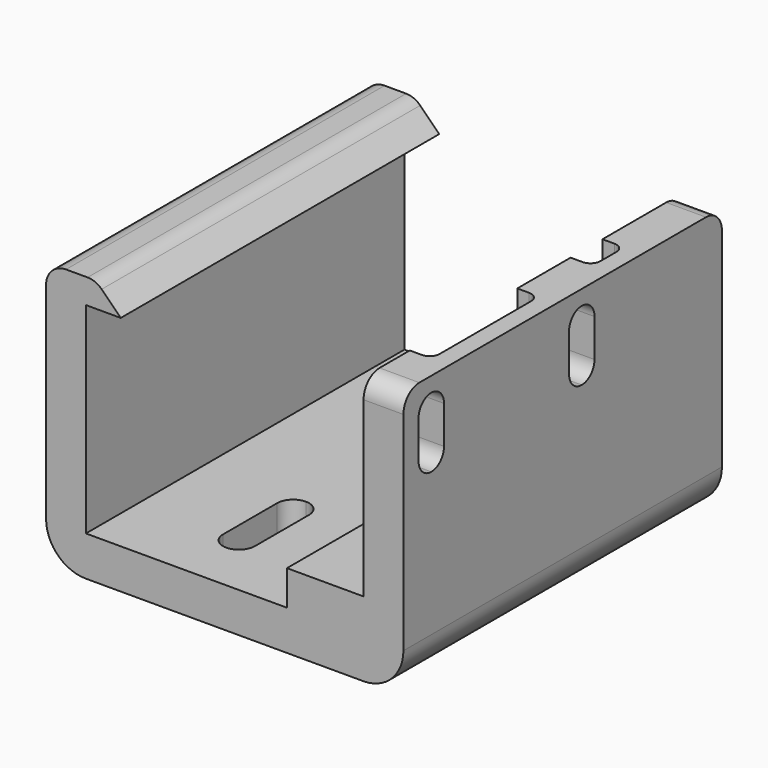
from build123d import *

# Parameters (mm, degrees)
F1_DEPTH  = 40
F2_R      = 4
F3_R      = 2
F4_W      = 3.2
F4_H      = 7
F5_DEPTH  = 4
F6_R      = 1.59999
F7_W      = 3.2
F7_H      = 10
F8_DEPTH  = 4
F9_R      = 1.59999
F10_W     = 2.2
F10_H     = 4
F10_H_2   = 13.5
F11_DEPTH = 17
F12_R     = 2
F13_R     = 1
F14_R     = 2


# Not quite as in the source:
# - a fillet or chamfer is up to 0.001 mm smaller than in the source, because OpenCascade refuses the exact size


with BuildPart() as f1:
    # F0 (on Front) → F1 (new body)
    with BuildSketch(Plane.XZ):
        Polygon((21.0562500745, -30.2744720221), (21.0562500745, -3.3744720221), (17.0562500745, -3.3744720221), (17.0562500745, -22.7744720221), (9.3562500745, -22.7744720221), (9.3562500745, -26.2744720221), (-10.8437499255, -26.2744720221), (-10.8437499255, -6.0744720221), (-7.3437499255, -6.0744720221), (-9.8437499255, -3.5744720221), (-14.8437499255, -3.5744720221), (-14.8437499255, -30.2744720221), align=None)
    extrude(amount=F1_DEPTH)

    # F2
    f2_edges = [f1.edges().sort_by_distance(p)[0] for p in [
        (-14.84375, -20, -30.274472),
        (21.05625, -20, -30.274472),
    ]]
    fillet(f2_edges, radius=F2_R)

    # F3
    f3_edges = [f1.edges().sort_by_distance(p)[0] for p in [
        (-9.84375, -20, -3.574472),
    ]]
    fillet(f3_edges, radius=F3_R)

    # F4 (on face) → F5 (cut, through all)
    with BuildSketch(Plane.YZ.offset(21.0562500745)):
        with Locations((-17.6, -8.3744720221)):
            Rectangle(F4_W, F4_H)
        with Locations((-36.5, -8.3744720221)):
            Rectangle(F4_W, F4_H)
    extrude(amount=-F5_DEPTH, mode=Mode.SUBTRACT)

    # F6 (radius 1.6 in the source; OpenCascade refuses exactly that, so slightly less here)
    f6_edges = [f1.edges().sort_by_distance(p)[0] for p in [
        (19.05625, -19.2, -4.874472),
        (19.05625, -16, -4.874472),
        (19.05625, -16, -11.874472),
        (19.05625, -19.2, -11.874472),
        (19.05625, -38.1, -11.874472),
        (19.05625, -34.9, -11.874472),
        (19.05625, -34.9, -4.874472),
        (19.05625, -38.1, -4.874472),
    ]]
    fillet(f6_edges, radius=F6_R)

    # F7 (on face) → F8 (cut, through all)
    with BuildSketch(Plane(origin=(0, 0, -30.2744720221), x_dir=(1, 0, 0), z_dir=(0, 0, -1))):
        with Locations((-0.500000006, 10)):
            Rectangle(F7_W, F7_H)
        with Locations((-0.7437499255, 30)):
            Rectangle(F7_W, F7_H)
    extrude(amount=-F8_DEPTH, mode=Mode.SUBTRACT)

    # F9 (radius 1.6 in the source; OpenCascade refuses exactly that, so slightly less here)
    f9_edges = [f1.edges().sort_by_distance(p)[0] for p in [
        (0.85625, -35, -28.274472),
        (-2.34375, -35, -28.274472),
        (-2.1, -15, -28.274472),
        (1.1, -15, -28.274472),
        (0.85625, -25, -28.274472),
        (1.1, -5, -28.274472),
        (-2.34375, -25, -28.274472),
        (-2.1, -5, -28.274472),
    ]]
    fillet(f9_edges, radius=F9_R)

    # F10 (on face) → F11 (cut)
    with BuildSketch(Plane.XY.offset(-3.3744720221)):
        with Locations((18.1562500745, -12)):
            Rectangle(F10_W, F10_H)
        with Locations((18.1562500745, -27.45)):
            Rectangle(F10_W, F10_H_2)
    extrude(amount=-F11_DEPTH, mode=Mode.SUBTRACT)

    # F12
    f12_edges = [f1.edges().sort_by_distance(p)[0] for p in [
        (19.05625, -40, -3.374472),
        (19.05625, 0, -3.374472),
    ]]
    fillet(f12_edges, radius=F12_R)

    # F13
    f13_edges = [f1.edges().sort_by_distance(p)[0] for p in [
        (19.25625, -14, -11.874472),
        (19.25625, -10, -11.874472),
        (19.25625, -20.7, -11.874472),
        (19.25625, -34.2, -11.874472),
    ]]
    fillet(f13_edges, radius=F13_R)

    # F14
    f14_edges = [f1.edges().sort_by_distance(p)[0] for p in [
        (-14.84375, -20, -3.574472),
    ]]
    fillet(f14_edges, radius=F14_R)


solid = f1.part
